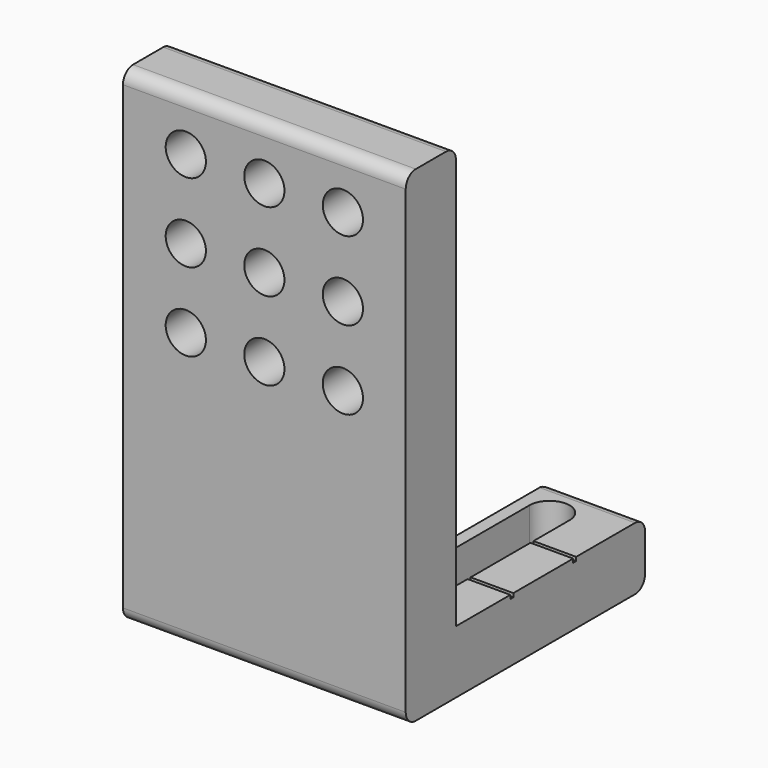
from build123d import *

# Parameters (mm, degrees)
F1_DEPTH  = 45
F3_DEPTH  = 10
F4_R      = 2
F5_R      = 3.2
F6_DEPTH  = 10
F2_W      = 14.6
F2_H      = 37.61
F7_DEPTH  = 10
F8_R      = 3
F9_R      = 1.99999
F2_W_2    = 6.8
F2_H_2    = 0.6
F10_DEPTH = 0.6


# Not quite as in the source:
# - a fillet or chamfer is up to 0.001 mm smaller than in the source, because OpenCascade refuses the exact size
# - a feature names something its author has since deleted; it is built from what else it names


with BuildPart() as f1:
    # F0 (on Right) → F1 (new body)
    with BuildSketch(Plane.YZ):
        Polygon((37.61, 0), (0, 0), (0, 67.3), (-10, 67.3), (-10, -10), (37.61, -10), align=None)
    extrude(amount=F1_DEPTH)

    # F2 (on face) → F3 (cut)
    with BuildSketch(Plane.XY):
        with BuildLine():
            Line((13.2, 6.11), (13.2, 31.11))
            ThreePointArc((13.2, 31.11), (10, 34.31), (6.8, 31.11))
            Line((6.8, 31.11), (6.8, 23.91))
            Line((6.8, 23.91), (6.8, 23.31))
            Line((6.8, 23.31), (6.8, 11.41))
            Line((6.8, 11.41), (6.8, 10.81))
            Line((6.8, 10.81), (6.8, 6.11))
            ThreePointArc((6.8, 6.11), (10, 2.91), (13.2, 6.11))
        make_face()
        with BuildLine():
            Line((38.2, 23.31), (38.2, 23.91))
            Line((38.2, 23.91), (38.2, 31.11))
            ThreePointArc((38.2, 31.11), (35, 34.31), (31.8, 31.11))
            Line((31.8, 31.11), (31.8, 6.11))
            ThreePointArc((31.8, 6.11), (35, 2.91), (38.2, 6.11))
            Line((38.2, 6.11), (38.2, 10.81))
            Line((38.2, 10.81), (38.2, 11.41))
            Line((38.2, 11.41), (38.2, 23.31))
        make_face()
    extrude(amount=-F3_DEPTH, mode=Mode.SUBTRACT)

    # F4
    f4_edges = [f1.edges().sort_by_distance(p)[0] for p in [
        (22.5, 37.61, -10),
        (22.5, -10, -10),
        (22.5, 0, 67.3),
        (22.5, -10, 67.3),
    ]]
    fillet(f4_edges, radius=F4_R)

    # F5 (on face) → F6 (cut)
    with BuildSketch(Plane.XZ.offset(10)):
        with Locations((10, 58.8)):
            Circle(F5_R)
        with Locations((22.5, 58.8)):
            Circle(F5_R)
        with Locations((35, 58.8)):
            Circle(F5_R)
        with Locations((35, 46.3)):
            Circle(F5_R)
        with Locations((22.5, 46.3)):
            Circle(F5_R)
        with Locations((10, 46.3)):
            Circle(F5_R)
        with Locations((10, 33.8)):
            Circle(F5_R)
        with Locations((22.5, 33.8)):
            Circle(F5_R)
        with Locations((35, 33.8)):
            Circle(F5_R)
    extrude(amount=-F6_DEPTH, mode=Mode.SUBTRACT)

    # F2 (on face) → F7 (cut)
    with BuildSketch(Plane.XY):
        with Locations((22.5, 18.805)):
            Rectangle(F2_W, F2_H)
    extrude(amount=-F7_DEPTH, mode=Mode.SUBTRACT)

    # F8
    f8_edges = [f1.edges().sort_by_distance(p)[0] for p in [
        (29.8, 0, -5),
        (15.2, 0, -5),
    ]]
    fillet(f8_edges, radius=F8_R)

    # F9 (radius 2 in the source; OpenCascade refuses exactly that, so slightly less here)
    f9_edges = [f1.edges().sort_by_distance(p)[0] for p in [
        (15.2, 37.61, -4),
        (15.2, 37.024214, -9.414214),
        (37.4, 37.61, 0),
        (7.6, 37.61, 0),
    ]]
    fillet(f9_edges, radius=F9_R)

    # F2 (on face) → F10 (cut)
    with BuildSketch(Plane.XY):
        with Locations((3.4, 11.11)):
            Rectangle(F2_W_2, F2_H_2)
        with Locations((3.4, 23.61)):
            Rectangle(F2_W_2, F2_H_2)
        with Locations((41.6, 11.11)):
            Rectangle(F2_W_2, F2_H_2)
        with Locations((41.6, 23.61)):
            Rectangle(F2_W_2, F2_H_2)
    extrude(amount=-F10_DEPTH, mode=Mode.SUBTRACT)


solid = f1.part
